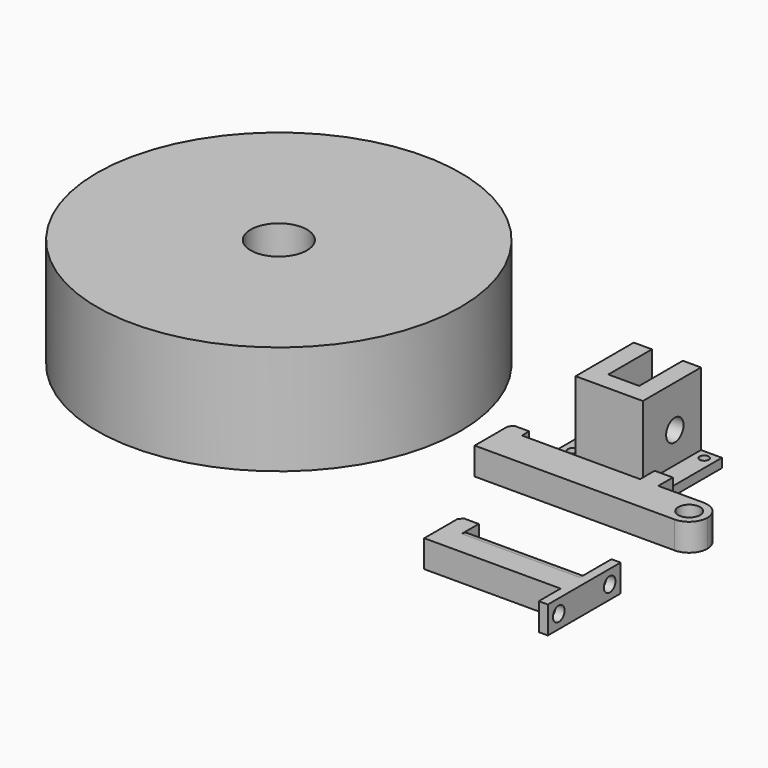
from build123d import *

# Parameters (mm, degrees)
F0_R      = 6
F1_DEPTH  = 15
F0_W      = 11.5
F0_H      = 40
F0_R_2    = 2.5
F0_W_2    = 17
F0_H_2    = 10
F0_H_3    = 30
F2_DEPTH  = 5
F3_DEPTH  = 40
F4_R      = 9.99999
F5_R      = 6
F6_DEPTH  = 52.2
F0_R_3    = 100
F0_R_4    = 15.5
F7_DEPTH  = 60
F0_W_3    = 5
F0_H_4    = 15
F0_H_5    = 20
F8_DEPTH  = 15
F9_R      = 4
F10_DEPTH = 25
F11_R     = 6.7597979746


# Not quite as in the source:
# - a fillet or chamfer is up to 0.001 mm smaller than in the source, because OpenCascade refuses the exact size


with BuildPart() as f1:
    # F0 (on Top) → F1 (new body)
    with BuildSketch(Plane.XY):
        Polygon((32.9961277544, 0), (-32.0038722456, 0), (-32.0038722456, 5), (-40.0256873742, 5), (-42.0038722456, 2.8751766719), (-42.0038722456, 0), (-42.0038722456, -20), (77.9961277544, -20), (77.9961277544, 0), (42.9961277544, 0), (42.9961277544, 10), (32.9961277544, 10), align=None)
        with Locations((67.9961277544, -10)):
            Circle(F0_R, mode=Mode.SUBTRACT)
    extrude(amount=F1_DEPTH)

    # F4 (radius 10 in the source; OpenCascade refuses exactly that, so slightly less here)
    f4_edges = [f1.edges().sort_by_distance(p)[0] for p in [
        (77.996128, 0, 7.5),
        (77.996128, -20, 7.5),
    ]]
    fillet(f4_edges, radius=F4_R)


with BuildPart() as f2:
    # F0 (on Top) → F2 (new body)
    with BuildSketch(Plane.XY):
        with Locations((-24.25, 40)):
            Rectangle(F0_W, F0_H)
        with Locations((-24.25, 25)):
            Circle(F0_R_2, mode=Mode.SUBTRACT)
        with Locations((-24.25, 55)):
            Circle(F0_R_2, mode=Mode.SUBTRACT)
        Polygon((-8.5, 30), (-8.5, 60), (-18.5, 60), (-18.5, 20), (-8.5, 20), align=None)
        with Locations((0, 25)):
            Rectangle(F0_W_2, F0_H_2)
        Polygon((18.5, 20), (18.5, 60), (8.5, 60), (8.5, 30), (8.5, 20), align=None)
        with Locations((24.25, 40)):
            Rectangle(F0_W, F0_H)
        with Locations((24.25, 25)):
            Circle(F0_R_2, mode=Mode.SUBTRACT)
        with Locations((24.25, 55)):
            Circle(F0_R_2, mode=Mode.SUBTRACT)
        with Locations((0, 45)):
            Rectangle(F0_W_2, F0_H_3)
    extrude(amount=-F2_DEPTH)

    # F0 (on Top) → F3 (join)
    with BuildSketch(Plane.XY):
        Polygon((-8.5, 30), (-8.5, 60), (-18.5, 60), (-18.5, 20), (-8.5, 20), align=None)
        Polygon((18.5, 20), (18.5, 60), (8.5, 60), (8.5, 30), (8.5, 20), align=None)
        with Locations((0, 25)):
            Rectangle(F0_W_2, F0_H_2)
    extrude(amount=F3_DEPTH)

    # F5 (on face) → F6 (cut)
    with BuildSketch(Plane.YZ.offset(18.5)):
        with Locations((42, 17)):
            Circle(F5_R)
    extrude(amount=-F6_DEPTH, mode=Mode.SUBTRACT)


with BuildPart() as f7:
    # F0 (on Top) → F7 (new body)
    with BuildSketch(Plane.XY):
        with Locations((-173.1806099415, 9.3010207638)):
            Circle(F0_R_3)
        with Locations((-173.1806099415, 9.3010207638)):
            Circle(F0_R_4, mode=Mode.SUBTRACT)
    extrude(amount=F7_DEPTH)


with BuildPart() as f8:
    # F0 (on Top) → F8 (new body)
    with BuildSketch(Plane.XY):
        Polygon((59.8999890685, -80.8080112338), (4.8999890685, -80.8080112338), (4.8999890685, -75.8080112338), (-3.1218260601, -75.8080112338), (-5.1000109315, -77.9328345619), (-5.1000109315, -80.8080112338), (-5.1000109315, -100.8080112338), (69.8999890685, -100.8080112338), (69.8999890685, -80.8080112338), align=None)
        Polygon((69.8999890685, -70.8080112338), (69.8999890685, -80.8080112338), (74.8999890685, -80.8080112338), (74.8999890685, -65.8080112338), (69.8999890685, -65.8080112338), align=None)
        with Locations((72.3999890685, -108.3080112338)):
            Rectangle(F0_W_3, F0_H_4)
        with Locations((72.3999890685, -90.8080112338)):
            Rectangle(F0_W_3, F0_H_5)
    extrude(amount=F8_DEPTH)

    # F9 (on face) → F10 (cut)
    with BuildSketch(Plane(origin=(69.8999890685, 0, 0), x_dir=(0, -1, 0), z_dir=(-1, 0, 0))):
        with Locations((73.3080112338, 7.5)):
            Circle(F9_R)
        with Locations((108.3080112338, 7.5)):
            Circle(F9_R)
    extrude(amount=-F10_DEPTH, mode=Mode.SUBTRACT)

    # F11
    f11_edges = [f8.edges().sort_by_distance(p)[0] for p in [
        (37.399989, -80.808011, 0),
        (37.399989, -80.808011, 15),
    ]]
    fillet(f11_edges, radius=F11_R)


solid = Compound([f1.part, f2.part, f7.part, f8.part])
